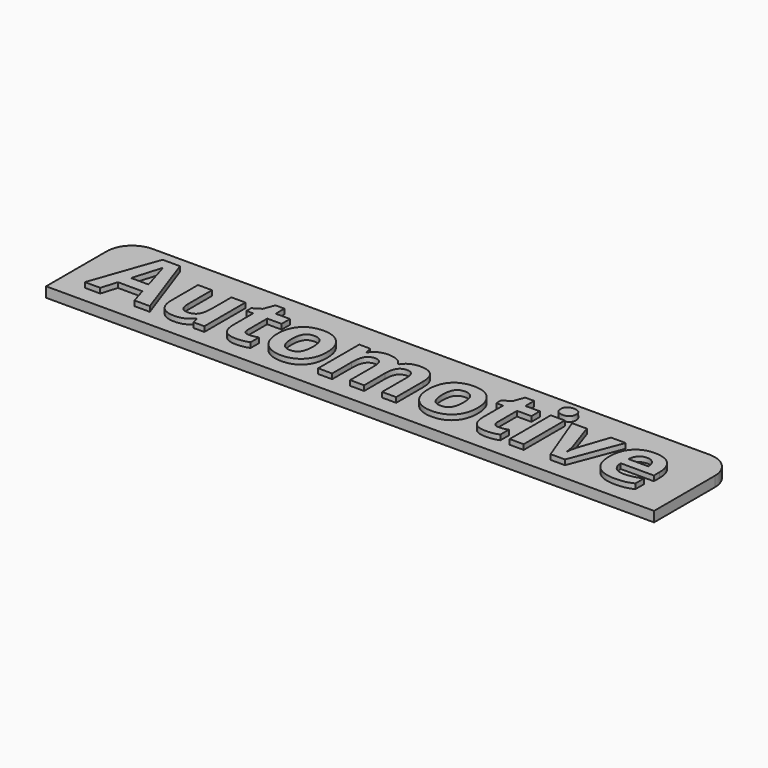
from build123d import *

# Parameters (mm, degrees)
F0_W         = 120
F0_H         = 20
F1_DEPTH     = 2
F2_TEXT_SIZE = 18.5737276733
F3_DEPTH     = 1
F4_R         = 5


# Not quite as in the source:
# - Text() gives the source's letters only with a copy of the font that has no kerning and outlines rounded to 1/6400 em; it was checked with that copy


with BuildPart() as f1:
    # F0 (on Top) → F1 (new body)
    with BuildSketch(Plane.XY):
        Rectangle(F0_W, F0_H)
    extrude(amount=F1_DEPTH)

    # F2 (on face) → F3 (join)
    with BuildSketch(Plane.XY.offset(2)):
        with Locations((-55, -6.6730839248)):
            Text('Automotive', F2_TEXT_SIZE, font='Open Sans', font_style=FontStyle.BOLD, text_align=(TextAlign.LEFT, TextAlign.BOTTOM))
    extrude(amount=F3_DEPTH)

    # F4
    f4_edges = [f1.edges().sort_by_distance(p)[0] for p in [
        (-60, 10, 1),
        (60, 10, 1),
    ]]
    fillet(f4_edges, radius=F4_R)


solid = f1.part
